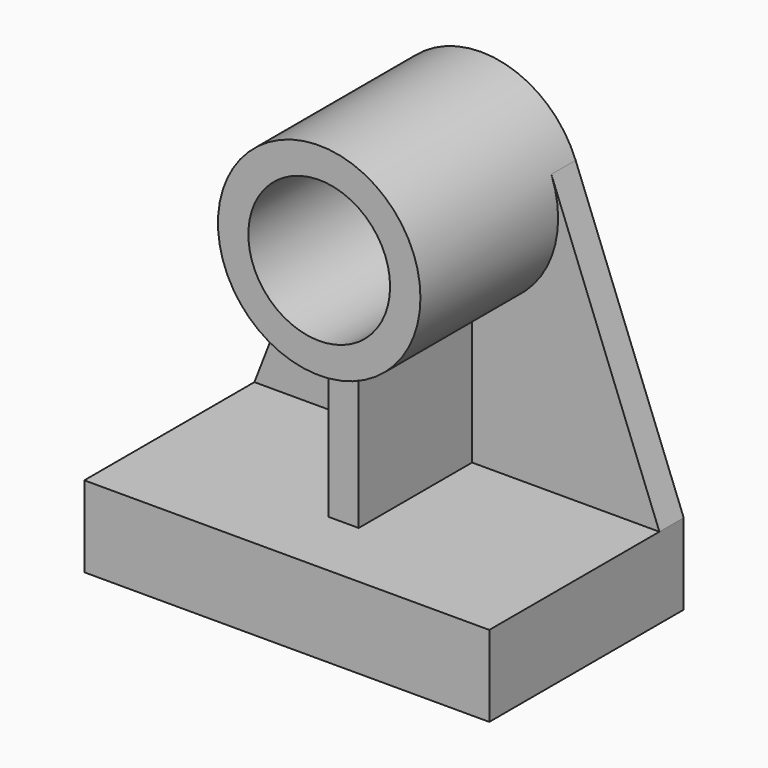
from build123d import *

# Parameters (mm, degrees)
F0_R     = 63.5
F0_R_2   = 44.45
F1_DEPTH = 127
F3_DEPTH = 19.05
F4_W     = 254
F4_H     = 50.8
F5_DEPTH = 152.4
F7_DEPTH = 88.9


with BuildPart() as f1:
    # F0 (on Front) → F1 (new body)
    with BuildSketch(Plane.XZ):
        Circle(F0_R)
        Circle(F0_R_2, mode=Mode.SUBTRACT)
    extrude(amount=F1_DEPTH)

    # F2 (on Front) → F3 (join)
    with BuildSketch(Plane.XZ):
        with BuildLine():
            Line((127, -152.4), (59.2277468166, 22.8981223472))
            ThreePointArc((59.2277468166, 22.8981223472), (52.3749977043, -35.904172675), (0, -63.5))
            Line((0, -63.5), (0, -152.4))
            Line((0, -152.4), (127, -152.4))
        make_face()
        with BuildLine():
            Line((0, -152.4), (0, -63.5))
            ThreePointArc((0, -63.5), (-52.3749977043, -35.904172675), (-59.2277468166, 22.8981223472))
            Line((-59.2277468166, 22.8981223472), (-127, -152.4))
            Line((-127, -152.4), (0, -152.4))
        make_face()
    extrude(amount=F3_DEPTH)

    # F4 (on face) → F5 (join)
    with BuildSketch(Plane(origin=(0, 0, 0), x_dir=(-1, 0, 0), z_dir=(0, 1, 0))):
        with Locations((0, -177.8)):
            Rectangle(F4_W, F4_H)
    extrude(amount=-F5_DEPTH)

    # F6 (on face) → F7 (join)
    with BuildSketch(Plane.XZ.offset(19.05)):
        with BuildLine():
            Line((0, -152.4), (0, -63.5))
            ThreePointArc((0, -63.5), (-4.776028159, -63.3201354628), (-9.525, -62.7815607882))
            Line((-9.525, -62.7815607882), (-9.525, -152.4))
            Line((-9.525, -152.4), (0, -152.4))
        make_face()
        with BuildLine():
            ThreePointArc((9.525, -62.7815607882), (4.776028159, -63.3201354628), (0, -63.5))
            Line((0, -63.5), (0, -152.4))
            Line((0, -152.4), (9.525, -152.4))
            Line((9.525, -152.4), (9.525, -62.7815607882))
        make_face()
    extrude(amount=F7_DEPTH)


solid = f1.part
